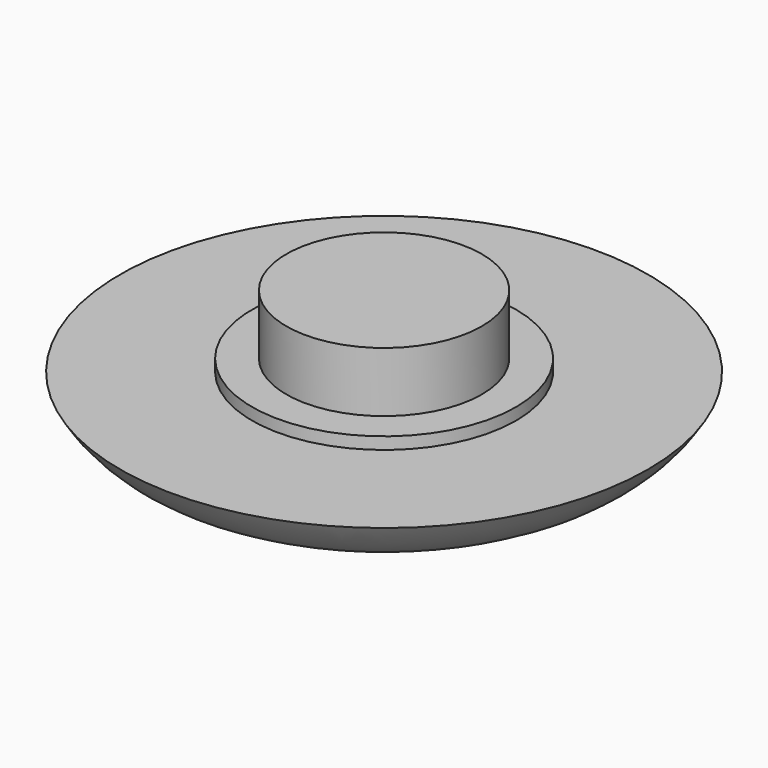
from build123d import *

# Parameters (mm, degrees)
F0_R     = 4.075
F1_DEPTH = 5.5
F0_R_2   = 11
F0_R_3   = 5.5
F2_DEPTH = 2.5
F3_DEPTH = 3


# Not quite as in the source:
# - a fillet or chamfer that OpenCascade refuses, or shapes differently, is made with other operations: its cross-section is extruded or revolved along the edge and cut away or added


with BuildPart() as f1:
    # F0 (on Top) → F1 (new body)
    with BuildSketch(Plane.XY):
        Circle(F0_R)
    extrude(amount=F1_DEPTH)


with BuildPart() as f2:
    # F0 (on Top) → F2 (new body)
    with BuildSketch(Plane.XY):
        Circle(F0_R_2)
        Circle(F0_R_3, mode=Mode.SUBTRACT)
    extrude(amount=F2_DEPTH)

    # F4: fillet of radius 5 on 1 edges, made by hand

    # F4_s1 → F4_t2 (revolve, cut)
    with BuildSketch(Plane.XZ):
        with BuildLine():
            ThreePointArc((11, 2.5), (9.1698729811, 0.6698729811), (6.6698729811, 0))
            Line((6.6698729811, 0), (11, 0))
            Line((11, 0), (11, 2.5))
        make_face()
    revolve(axis=Axis((0, 0, 0), (0, 0, 1)), mode=Mode.SUBTRACT)


with BuildPart() as f3:
    # F0 (on Top) → F3 (new body)
    with BuildSketch(Plane.XY):
        Circle(F0_R_3)
        Circle(F0_R, mode=Mode.SUBTRACT)
    extrude(amount=F3_DEPTH)


solid = Compound([f1.part, f2.part, f3.part])
